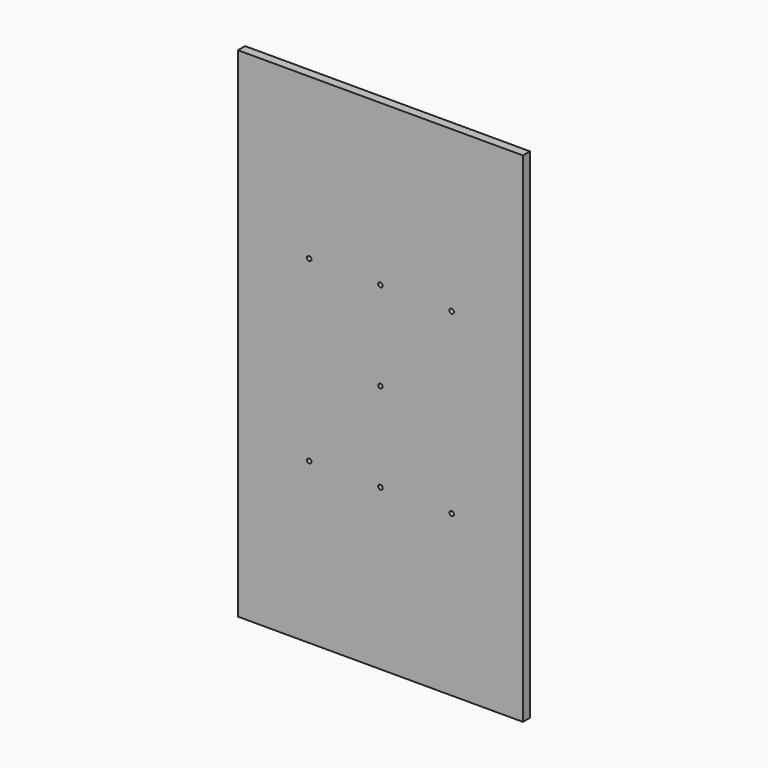
from build123d import *

# Parameters (mm, degrees)
F0_W     = 203.2
F0_H     = 355.6
F1_DEPTH = 6.35
F3_DEPTH = 25.4


# Not quite as in the source:
# - a feature names something its author has since deleted; it is built from what else it names


with BuildPart() as f1:
    # F0 (on Front) → F1 (new body)
    with BuildSketch(Plane.XZ):
        with Locations((-1.7359743744, 100.030120313)):
            Rectangle(F0_W, F0_H)
    extrude(amount=F1_DEPTH)

    # F2 (on face) → F3 (cut)
    with BuildSketch(Plane.XZ.offset(6.35)):
        with BuildLine():
            Line((-1.7359743744, 100.030120313), (-0.1484743744, 100.030120313))
            ThreePointArc((-0.1484743744, 100.030120313), (-0.6134423593, 101.1526523282), (-1.7359743744, 101.617620313))
            Line((-1.7359743744, 101.617620313), (-1.7359743744, 100.030120313))
        make_face()
        with BuildLine():
            ThreePointArc((-1.7359743744, 98.442620313), (-0.6134423593, 98.9075882979), (-0.1484743744, 100.030120313))
            Line((-0.1484743744, 100.030120313), (-1.7359743744, 100.030120313))
            Line((-1.7359743744, 100.030120313), (-1.7359743744, 98.442620313))
        make_face()
        with BuildLine():
            Line((-1.7359743744, 100.030120313), (-1.7359743744, 101.617620313))
            ThreePointArc((-1.7359743744, 101.617620313), (-2.8585063895, 101.1526523282), (-3.3234743744, 100.030120313))
            Line((-3.3234743744, 100.030120313), (-1.7359743744, 100.030120313))
        make_face()
        with BuildLine():
            ThreePointArc((-3.3234743744, 100.030120313), (-2.8585063895, 98.9075882979), (-1.7359743744, 98.442620313))
            Line((-1.7359743744, 98.442620313), (-1.7359743744, 100.030120313))
            Line((-1.7359743744, 100.030120313), (-3.3234743744, 100.030120313))
        make_face()
        with BuildLine():
            Line((-1.7359743744, 163.530120313), (-1.7359743744, 161.942620313))
            ThreePointArc((-1.7359743744, 161.942620313), (-0.6134423593, 162.4075882979), (-0.1484743744, 163.530120313))
            Line((-0.1484743744, 163.530120313), (-1.7359743744, 163.530120313))
        make_face()
        with BuildLine():
            ThreePointArc((-3.3234743744, 163.530120313), (-2.8585063895, 162.4075882979), (-1.7359743744, 161.942620313))
            Line((-1.7359743744, 161.942620313), (-1.7359743744, 163.530120313))
            Line((-1.7359743744, 163.530120313), (-3.3234743744, 163.530120313))
        make_face()
        with BuildLine():
            Line((-1.7359743744, 36.530120313), (-1.7359743744, 38.117620313))
            ThreePointArc((-1.7359743744, 38.117620313), (-2.8585063895, 37.6526523282), (-3.3234743744, 36.530120313))
            Line((-3.3234743744, 36.530120313), (-1.7359743744, 36.530120313))
        make_face()
        with BuildLine():
            ThreePointArc((-0.1484743744, 36.530120313), (-0.6134423593, 37.6526523282), (-1.7359743744, 38.117620313))
            Line((-1.7359743744, 38.117620313), (-1.7359743744, 36.530120313))
            Line((-1.7359743744, 36.530120313), (-0.1484743744, 36.530120313))
        make_face()
        with BuildLine():
            ThreePointArc((-1.7359743744, 165.117620313), (-2.8585063895, 164.6526523282), (-3.3234743744, 163.530120313))
            Line((-3.3234743744, 163.530120313), (-1.7359743744, 163.530120313))
            Line((-1.7359743744, 163.530120313), (-1.7359743744, 165.117620313))
        make_face()
        with BuildLine():
            Line((-1.7359743744, 163.530120313), (-0.1484743744, 163.530120313))
            ThreePointArc((-0.1484743744, 163.530120313), (-0.6134423593, 164.6526523282), (-1.7359743744, 165.117620313))
            Line((-1.7359743744, 165.117620313), (-1.7359743744, 163.530120313))
        make_face()
        with BuildLine():
            ThreePointArc((-1.7359743744, 34.942620313), (-0.6134423593, 35.4075882979), (-0.1484743744, 36.530120313))
            Line((-0.1484743744, 36.530120313), (-1.7359743744, 36.530120313))
            Line((-1.7359743744, 36.530120313), (-1.7359743744, 34.942620313))
        make_face()
        with BuildLine():
            Line((-1.7359743744, 36.530120313), (-3.3234743744, 36.530120313))
            ThreePointArc((-3.3234743744, 36.530120313), (-2.8585063895, 35.4075882979), (-1.7359743744, 34.942620313))
            Line((-1.7359743744, 34.942620313), (-1.7359743744, 36.530120313))
        make_face()
        with BuildLine():
            Line((49.0640256256, 36.530120313), (50.6515256256, 36.530120313))
            ThreePointArc((50.6515256256, 36.530120313), (49.0640256256, 38.117620313), (47.4765256256, 36.530120313))
            Line((47.4765256256, 36.530120313), (49.0640256256, 36.530120313))
        make_face()
        with BuildLine():
            ThreePointArc((47.4765256256, 36.530120313), (49.0640256256, 34.942620313), (50.6515256256, 36.530120313))
            Line((50.6515256256, 36.530120313), (49.0640256256, 36.530120313))
            Line((49.0640256256, 36.530120313), (47.4765256256, 36.530120313))
        make_face()
        with BuildLine():
            Line((49.0640256256, 163.530120313), (50.6515256256, 163.530120313))
            ThreePointArc((50.6515256256, 163.530120313), (49.0640256256, 165.117620313), (47.4765256256, 163.530120313))
            Line((47.4765256256, 163.530120313), (49.0640256256, 163.530120313))
        make_face()
        with BuildLine():
            ThreePointArc((47.4765256256, 163.530120313), (49.0640256256, 161.942620313), (50.6515256256, 163.530120313))
            Line((50.6515256256, 163.530120313), (49.0640256256, 163.530120313))
            Line((49.0640256256, 163.530120313), (47.4765256256, 163.530120313))
        make_face()
        with BuildLine():
            Line((-52.5359743744, 163.530120313), (-50.9484743744, 163.530120313))
            ThreePointArc((-50.9484743744, 163.530120313), (-52.5359743744, 165.117620313), (-54.1234743744, 163.530120313))
            Line((-54.1234743744, 163.530120313), (-52.5359743744, 163.530120313))
        make_face()
        with BuildLine():
            ThreePointArc((-54.1234743744, 163.530120313), (-52.5359743744, 161.942620313), (-50.9484743744, 163.530120313))
            Line((-50.9484743744, 163.530120313), (-52.5359743744, 163.530120313))
            Line((-52.5359743744, 163.530120313), (-54.1234743744, 163.530120313))
        make_face()
        with BuildLine():
            Line((-52.5359743744, 36.530120313), (-50.9484743744, 36.530120313))
            ThreePointArc((-50.9484743744, 36.530120313), (-52.5359743744, 38.117620313), (-54.1234743744, 36.530120313))
            Line((-54.1234743744, 36.530120313), (-52.5359743744, 36.530120313))
        make_face()
        with BuildLine():
            ThreePointArc((-54.1234743744, 36.530120313), (-52.5359743744, 34.942620313), (-50.9484743744, 36.530120313))
            Line((-50.9484743744, 36.530120313), (-52.5359743744, 36.530120313))
            Line((-52.5359743744, 36.530120313), (-54.1234743744, 36.530120313))
        make_face()
    extrude(amount=-F3_DEPTH, mode=Mode.SUBTRACT)


solid = f1.part
